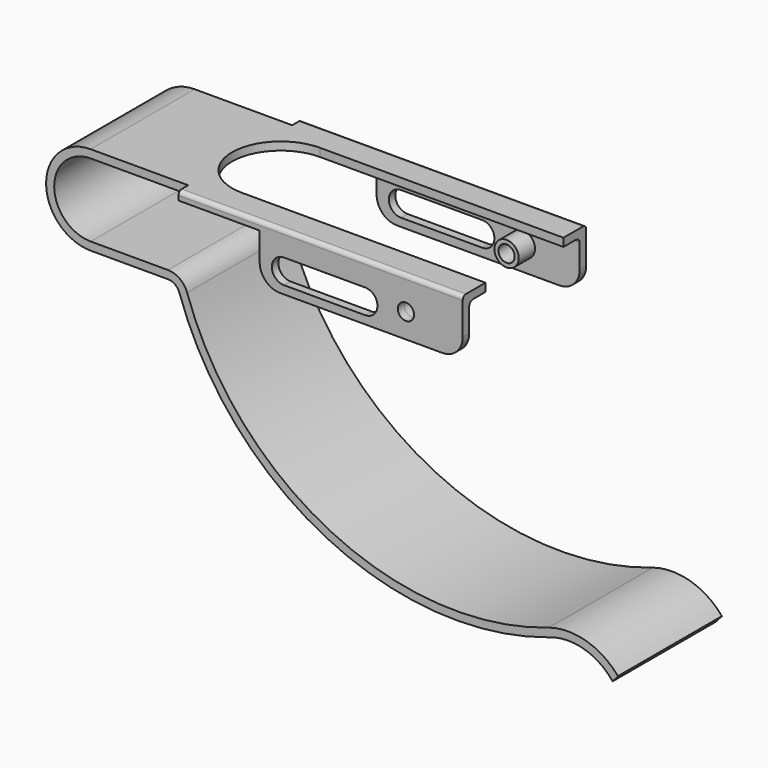
from build123d import *

# Parameters (mm, degrees)
F1_DEPTH  = 16
F2_W      = 70
F2_H      = 3
F3_DEPTH  = 2.1
F4_W      = 50
F4_H      = 14
F5_DEPTH  = 2
F6_R      = 0.99999
F9_DEPTH  = 2
F11_DEPTH = 38.001
F13_D     = 4
F14_R     = 3
F14_R_2   = 2
F15_DEPTH = 5
F16_R     = 5


# Not quite as in the source:
# - a fillet or chamfer is up to 0.001 mm smaller than in the source, because OpenCascade refuses the exact size
# - a pattern or mirror of a feature is missing from the dataset's text; its kind, count and spacing are read off the source's solid


with BuildPart() as f1:
    # F0 (on Front) → F1 (new body)
    with BuildSketch(Plane.XZ):
        with BuildLine():
            ThreePointArc((0, -9), (-9, 0), (0, 9))
            Line((0, 9), (94, 9))
            Line((94, 9), (94, 11))
            Line((94, 11), (0, 11))
            ThreePointArc((0, 11), (-11, 0), (0, -11))
            Line((0, -11), (19, -11))
            ThreePointArc((19, -11), (20.7464347921, -11.5607448848), (21.84, -13.0333563221))
            ThreePointArc((21.84, -13.0333563221), (57.9725997897, -54.3183684737), (112.7014609544, -58.1613818136))
            ThreePointArc((112.7014609544, -58.1613818136), (121.3224001133, -57.7984242203), (128.5187831367, -62.5591386181))
            Line((128.5187831367, -62.5591386181), (129.8270557762, -61))
            ThreePointArc((129.8270557762, -61), (122.0920530207, -55.9384698962), (112.8483757943, -56))
            ThreePointArc((112.8483757943, -56), (59.2303979034, -52.7086373708), (23.7333333333, -12.3889272035))
            ThreePointArc((23.7333333333, -12.3889272035), (21.9107246536, -9.9345748081), (19, -9))
            Line((19, -9), (0, -9))
        make_face()
    extrude(amount=F1_DEPTH)

    # F2 (on face) → F3 (join)
    with BuildSketch(Plane.XY.offset(11)):
        with Locations((59, -17.5)):
            Rectangle(F2_W, F2_H)
    extrude(amount=-F3_DEPTH)

    # F4 (on face) → F5 (join)
    with BuildSketch(Plane.XZ.offset(19)):
        with Locations((69, 4)):
            Rectangle(F4_W, F4_H)
    extrude(amount=-F5_DEPTH)

    # F6 (radius 1 in the source; OpenCascade refuses exactly that, so slightly less here)
    f6_edges = [f1.edges().sort_by_distance(p)[0] for p in [
        (59, -19, 11),
        (69, -17, 8.9),
    ]]
    fillet(f6_edges, radius=F6_R)

    # F7: F1 across plane


with BuildPart() as f1_1:
    add(f1.part)
    add(f1.part.mirror(Plane.XZ))

    # F8 (on face) → F9 (cut)
    with BuildSketch(Plane.XY.offset(11)):
        with BuildLine():
            Line((94, 12), (34, 12))
            ThreePointArc((34, 12), (22, 0), (34, -12))
            Line((34, -12), (94, -12))
            Line((94, -12), (94, 12))
        make_face()
    extrude(amount=-F9_DEPTH, mode=Mode.SUBTRACT)

    # F10 (on face) → F11 (cut, through all)
    with BuildSketch(Plane.XZ.offset(19)):
        with BuildLine():
            ThreePointArc((50, 5), (47, 2), (50, -1))
            Line((50, -1), (70, -1))
            ThreePointArc((70, -1), (73, 2), (70, 5))
            Line((70, 5), (50, 5))
        make_face()
    extrude(amount=-F11_DEPTH, mode=Mode.SUBTRACT)

    # F13 (through all)
    with Locations(Plane.XZ.offset(19)):
        with Locations((80, 3)):
            Hole(F13_D / 2)

    # F14 (on face) → F15 (join)
    with BuildSketch(Plane(origin=(0, -17, 0), x_dir=(-1, 0, 0), z_dir=(0, 1, 0))):
        with Locations((-80, 3)):
            Circle(F14_R)
        with Locations((-80, 3)):
            Circle(F14_R_2, mode=Mode.SUBTRACT)
    f15 = extrude(amount=F15_DEPTH)

    # F15_copies: F15 across plane
    add(f15.mirror(Plane.ZX))

    # F16
    f16_edges = [f1_1.edges().sort_by_distance(p)[0] for p in [
        (94, -18, -3),
        (94, 18, -3),
        (44, -18, -3),
        (44, 18, -3),
    ]]
    fillet(f16_edges, radius=F16_R)


solid = f1_1.part
